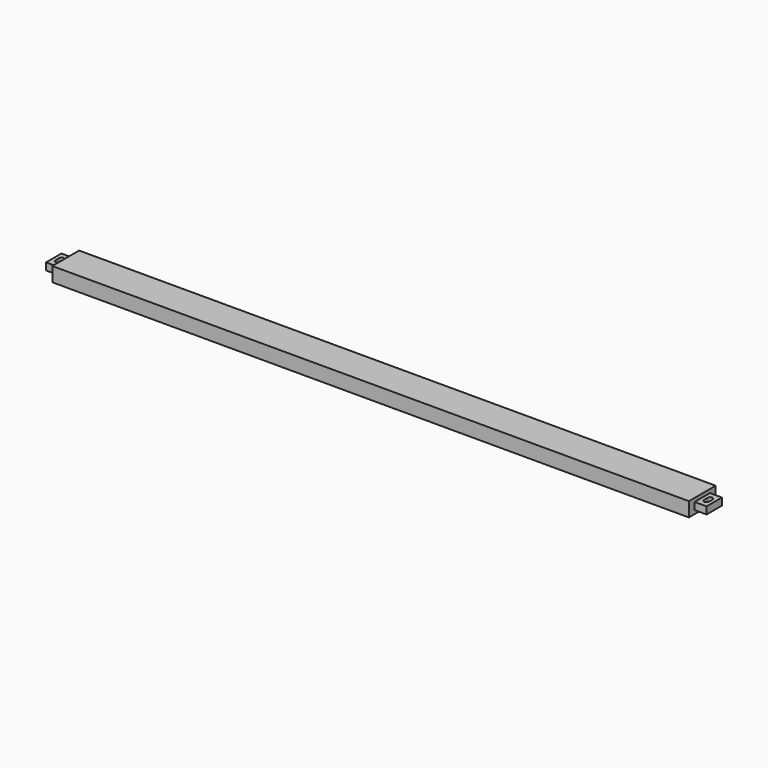
from build123d import *

# Parameters (mm, degrees)
F0_W     = 88.9
F0_H     = 38.1
F1_DEPTH = 1752.6
F3_W     = 88.9
F3_H     = 38.1
F3_W_2   = 50.8
F3_H_2   = 19.05
F4_DEPTH = 31.75
F6_DEPTH = 28.576


# Not quite as in the source:
# - a pattern or mirror of a feature is missing from the dataset's text; its kind, count and spacing are read off the source's solid


with BuildPart() as f1:
    # F0 (on Right) → F1 (new body)
    with BuildSketch(Plane.YZ):
        Rectangle(F0_W, F0_H)
    extrude(amount=F1_DEPTH)

    # F3 (on face) → F4 (cut)
    with BuildSketch(Plane(origin=(0, 0, 0), x_dir=(0, -1, 0), z_dir=(-1, 0, 0))):
        Rectangle(F3_W, F3_H)
        Rectangle(F3_W_2, F3_H_2, mode=Mode.SUBTRACT)
    f4 = extrude(amount=-F4_DEPTH, mode=Mode.SUBTRACT)

    # F4_copies: F4 across plane
    add(f4.mirror(Plane(origin=(876.3, 0, 0), x_dir=(0, 0, 1), z_dir=(1, 0, 0))), mode=Mode.SUBTRACT)

    # F5 (on face) → F6 (cut, through all)
    with BuildSketch(Plane.XY.offset(9.525)):
        with BuildLine():
            Line((9.525, 6.35), (9.525, -6.35))
            ThreePointArc((9.525, -6.35), (15.875, -12.7), (22.225, -6.35))
            Line((22.225, -6.35), (22.225, 6.35))
            ThreePointArc((22.225, 6.35), (15.875, 12.7), (9.525, 6.35))
        make_face()
    f6 = extrude(amount=-F6_DEPTH, mode=Mode.SUBTRACT)

    # F6_copies: F6 across plane
    add(f6.mirror(Plane(origin=(876.3, 0, 0), x_dir=(0, 0, 1), z_dir=(1, 0, 0))), mode=Mode.SUBTRACT)


solid = f1.part
